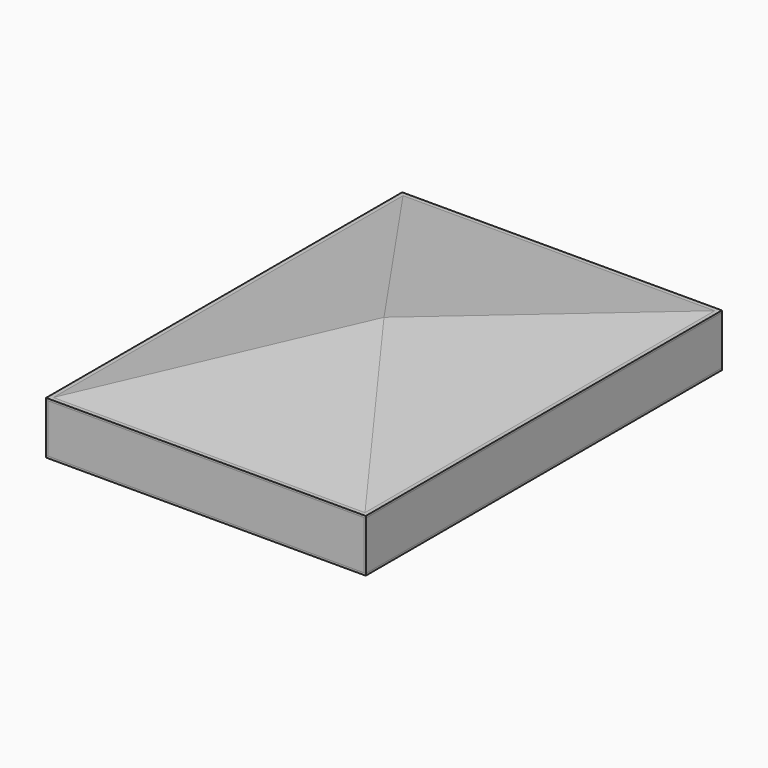
from build123d import *

# Parameters (mm, degrees)
F0_W      = 501.65
F0_H      = 698.5
F0_W_2    = 450.85
F0_H_2    = 647.7
F0_W_3    = 374.65
F0_H_3    = 571.5
F1_DEPTH  = 3.175
F2_W      = 3.175
F2_H      = 698.5
F3_DEPTH  = 76.2
F5_W      = 495.3
F5_H      = 3.175
F6_DEPTH  = 76.2
F8_W      = 501.65
F8_H      = 698.5
F8_W_2    = 488.95
F8_H_2    = 685.8
F9_DEPTH  = 3.175
F11_DEPTH = 685.8
F13_DEPTH = 501.651


# Not quite as in the source:
# - a pattern or mirror of a feature is missing from the dataset's text; its kind, count and spacing are read off the source's solid
# - a feature names something its author has since deleted; it is built from what else it names


with BuildPart() as f1:
    # F0 (on Top) → F1 (new body)
    with BuildSketch(Plane.XY):
        Rectangle(F0_W, F0_H)
        Rectangle(F0_W_2, F0_H_2, mode=Mode.SUBTRACT)
        Rectangle(F0_W_2, F0_H_2)
        Rectangle(F0_W_3, F0_H_3, mode=Mode.SUBTRACT)
    extrude(amount=F1_DEPTH)


with BuildPart() as f3:
    # F2 (on face) → F3 (new body)
    with BuildSketch(Plane.XY.offset(3.175)):
        with Locations((-249.2375, 0)):
            Rectangle(F2_W, F2_H)
    extrude(amount=F3_DEPTH)


with BuildPart() as f4_1:
    # F4: instance of F3
    add(f3.part.mirror(Plane.YZ))


with BuildPart() as f6:
    # F5 (on face) → F6 (new body, through all)
    with BuildSketch(Plane.XY.offset(3.175)):
        with Locations((0, -347.6625)):
            Rectangle(F5_W, F5_H)
    extrude(amount=F6_DEPTH)


with BuildPart() as f7_1:
    # F7: instance of F6
    add(f6.part.mirror(Plane.XZ))


with BuildPart() as f9:
    # F8 (on face) → F9 (new body)
    with BuildSketch(Plane.XY.offset(79.375)):
        Rectangle(F8_W, F8_H)
        Rectangle(F8_W_2, F8_H_2, mode=Mode.SUBTRACT)
    extrude(amount=F9_DEPTH)


with BuildPart() as f11:
    # F10 (on face) → F11 (new body, through all)
    with BuildSketch(Plane.XZ.offset(-342.9)):
        Polygon((0, 133.35), (-244.475, 82.55), (0, 82.55), align=None)
        Polygon((244.475, 82.55), (0, 133.35), (0, 82.55), align=None)
    extrude(amount=F11_DEPTH)

    # F12 (on face) → F13 (cut, through all)
    with BuildSketch(Plane.YZ.offset(250.825)):
        Polygon((0, 133.35), (342.9, 82.55), (342.9, 133.35), align=None)
    f13 = extrude(amount=-F13_DEPTH, mode=Mode.SUBTRACT)

    # F13_copies: F13 across plane
    add(f13.mirror(Plane(origin=(0, 0, 0), x_dir=(0, 0, -1), z_dir=(0, -1, 0))), mode=Mode.SUBTRACT)


solid = Compound([f1.part, f3.part, f4_1.part, f6.part, f7_1.part, f9.part, f11.part])
